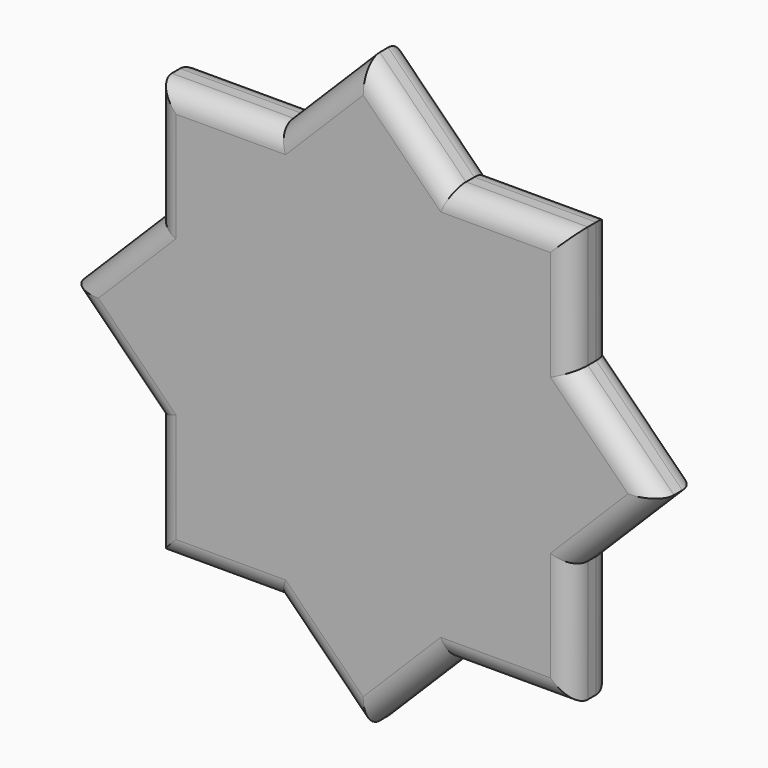
from build123d import *

# Parameters (mm, degrees)
F1_DEPTH     = 6.35
F2_TEXT_SIZE = 4.3392533011
F3_DEPTH     = 2.54
F4_R         = 2.54


# Not quite as in the source:
# - the program builds the solid bodies; features that only make, move or delete a surface that nothing else refers to are left out
# - Text() gives the source's letters only with a copy of the font that has no kerning and outlines rounded to 1/6400 em; it was checked with that copy


with BuildPart() as f1:
    # F0 (on Front) → F1 (new body)
    with BuildSketch(Plane.XZ):
        Polygon((-25.4, -10.5210244843), (-25.4, -25.4), (-10.5210244843, -25.4), align=None)
        Polygon((-25.4, -10.5210244843), (-10.5210244843, -25.4), (10.5210244843, -25.4), (25.4, -10.5210244843), (25.4, 10.5210244843), (10.5210244843, 25.4), (-10.5210244843, 25.4), (-25.4, 10.5210244843), align=None)
        Polygon((10.5210244843, -25.4), (-10.5210244843, -25.4), (0, -35.9210244843), align=None)
        Polygon((-35.9210244843, 0), (-25.4, -10.5210244843), (-25.4, 10.5210244843), align=None)
        Polygon((25.4, -10.5210244843), (10.5210244843, -25.4), (25.4, -25.4), align=None)
        Polygon((-25.4, 25.4), (-25.4, 10.5210244843), (-10.5210244843, 25.4), align=None)
        Polygon((25.4, 10.5210244843), (25.4, -10.5210244843), (35.9210244843, 0), align=None)
        Polygon((0, 35.9210244843), (-10.5210244843, 25.4), (10.5210244843, 25.4), align=None)
        Polygon((10.5210244843, 25.4), (25.4, 10.5210244843), (25.4, 25.4), align=None)
    extrude(amount=F1_DEPTH)

    # F2 (on face) → F3 (join)
    with BuildSketch(Plane(origin=(0, 0, 0), x_dir=(-1, 0, 0), z_dir=(0, 1, 0))):
        with Locations((-19.2311477271, -2.2271409272)):
            Text('Happy fathers day', F2_TEXT_SIZE, font='Open Sans', font_style=FontStyle.BOLDITALIC, text_align=(TextAlign.LEFT, TextAlign.BOTTOM))
        with Locations((-7.9558692276, -8.1285254167)):
            Text('dad!!!!', F2_TEXT_SIZE, font='Open Sans', font_style=FontStyle.BOLDITALIC, text_align=(TextAlign.LEFT, TextAlign.BOTTOM))
    extrude(amount=F3_DEPTH)

    # F4
    f4_edges = [f1.edges().sort_by_distance(p)[0] for p in [
        (17.960512, 0, 25.4),
        (5.260512, 0, 30.660512),
        (-5.260512, 0, 30.660512),
        (-17.960512, 0, 25.4),
        (-25.4, 0, 17.960512),
        (-30.660512, 0, 5.260512),
        (-30.660512, 0, -5.260512),
        (-25.4, 0, -17.960512),
        (-17.960512, 0, -25.4),
        (-5.260512, 0, -30.660512),
        (5.260512, 0, -30.660512),
        (17.960512, 0, -25.4),
        (25.4, 0, -17.960512),
        (30.660512, 0, -5.260512),
        (30.660512, 0, 5.260512),
        (25.4, 0, 17.960512),
        (-30.660512, -6.35, 5.260512),
        (-17.960512, -6.35, -25.4),
        (-5.260512, -6.35, -30.660512),
        (5.260512, -6.35, -30.660512),
        (17.960512, -6.35, -25.4),
        (25.4, -6.35, -17.960512),
        (30.660512, -6.35, -5.260512),
        (30.660512, -6.35, 5.260512),
        (25.4, -6.35, 17.960512),
        (17.960512, -6.35, 25.4),
        (5.260512, -6.35, 30.660512),
        (-5.260512, -6.35, 30.660512),
        (-17.960512, -6.35, 25.4),
        (-25.4, -6.35, 17.960512),
        (-30.660512, -6.35, -5.260512),
        (-25.4, -6.35, -17.960512),
    ]]
    fillet(f4_edges, radius=F4_R)


solid = f1.part
